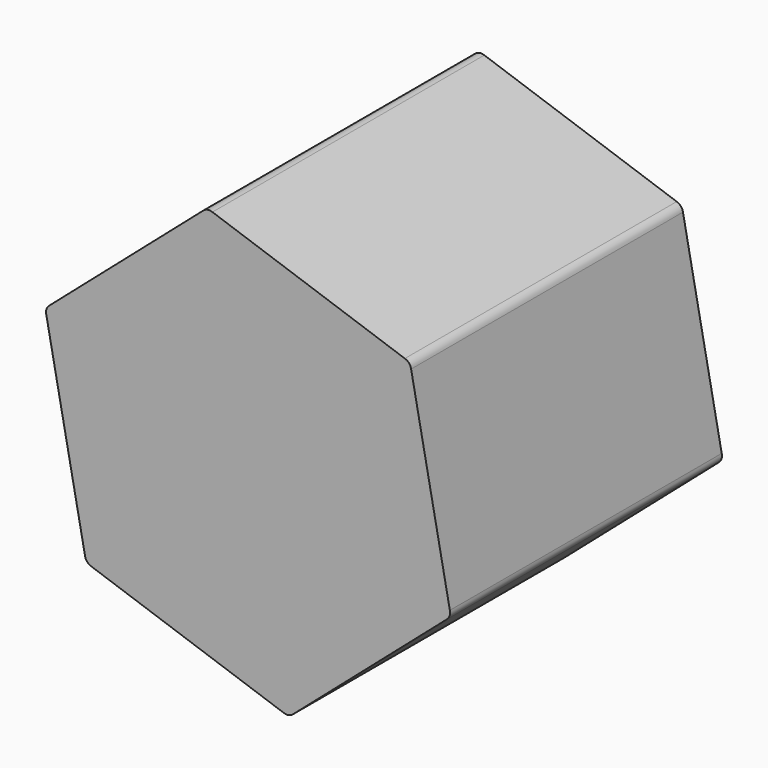
from build123d import *

# Parameters (mm, degrees)
F1_DEPTH    = 45.212
F2_T1_DEPTH = 97.7563484187


# Not quite as in the source:
# - a fillet or chamfer that OpenCascade refuses, or shapes differently, is made with other operations: its cross-section is extruded or revolved along the edge and cut away or added


with BuildPart() as f1:
    # F0 (on Front) → F1 (new body, symmetric)
    with BuildSketch(Plane.XZ):
        Polygon((53.9703455338, -18.609975213), (43.1018840651, 37.4347026768), (-10.8684614687, 56.0446778898), (-53.9703455338, 18.609975213), (-43.1018840651, -37.4347026768), (10.8684614687, -56.0446778898), align=None)
    extrude(amount=F1_DEPTH, both=True)

    # F2: fillet of radius 2.54 on 6 edges, made by hand

    # F2_s2 → F2_t1 (cut)
    with BuildSketch(Plane.XZ.offset(-48.8781742094)):
        with BuildLine():
            add(Edge.make_bspline(
                [(-11.9756422622, 55.0830729689), (-10.8684614687, 56.0446778898), (-9.4820967821, 55.5666336564)],
                knots=[0, 0, 0, 1, 1, 1], degree=2, weights=[1, 1, 1]))
            Line((-9.4820967821, 55.5666336564), (-10.8684614687, 56.0446778898))
            Line((-10.8684614687, 56.0446778898), (-11.9756422622, 55.0830729689))
        make_face()
        with BuildLine():
            add(Edge.make_bspline(
                [(43.3810679582, 35.9950535226), (43.1018840651, 37.4347026768), (41.7155193785, 37.9127469102)],
                knots=[0, 0, 0, 1, 1, 1], degree=2, weights=[1, 1, 1]))
            Line((41.7155193785, 37.9127469102), (43.1018840651, 37.4347026768))
            Line((43.1018840651, 37.4347026768), (43.3810679582, 35.9950535226))
        make_face()
        with BuildLine():
            add(Edge.make_bspline(
                [(-53.6911616407, 17.1703260588), (-53.9703455338, 18.609975213), (-52.8631647403, 19.5715801338)],
                knots=[0, 0, 0, 1, 1, 1], degree=2, weights=[1, 1, 1]))
            Line((-52.8631647403, 19.5715801338), (-53.9703455338, 18.609975213))
            Line((-53.9703455338, 18.609975213), (-53.6911616407, 17.1703260588))
        make_face()
        with BuildLine():
            add(Edge.make_bspline(
                [(-41.7155193785, -37.9127469102), (-43.1018840651, -37.4347026768), (-43.3810679582, -35.9950535226)],
                knots=[0, 0, 0, 1, 1, 1], degree=2, weights=[1, 1, 1]))
            Line((-43.3810679582, -35.9950535226), (-43.1018840651, -37.4347026768))
            Line((-43.1018840651, -37.4347026768), (-41.7155193785, -37.9127469102))
        make_face()
        with BuildLine():
            add(Edge.make_bspline(
                [(11.9756422622, -55.0830729689), (10.8684614687, -56.0446778898), (9.4820967821, -55.5666336564)],
                knots=[0, 0, 0, 1, 1, 1], degree=2, weights=[1, 1, 1]))
            Line((9.4820967821, -55.5666336564), (10.8684614687, -56.0446778898))
            Line((10.8684614687, -56.0446778898), (11.9756422622, -55.0830729689))
        make_face()
        with BuildLine():
            add(Edge.make_bspline(
                [(53.6911616407, -17.1703260588), (53.9703455338, -18.609975213), (52.8631647403, -19.5715801338)],
                knots=[0, 0, 0, 1, 1, 1], degree=2, weights=[1, 1, 1]))
            Line((52.8631647403, -19.5715801338), (53.9703455338, -18.609975213))
            Line((53.9703455338, -18.609975213), (53.6911616407, -17.1703260588))
        make_face()
    extrude(amount=F2_T1_DEPTH, mode=Mode.SUBTRACT)


solid = f1.part
